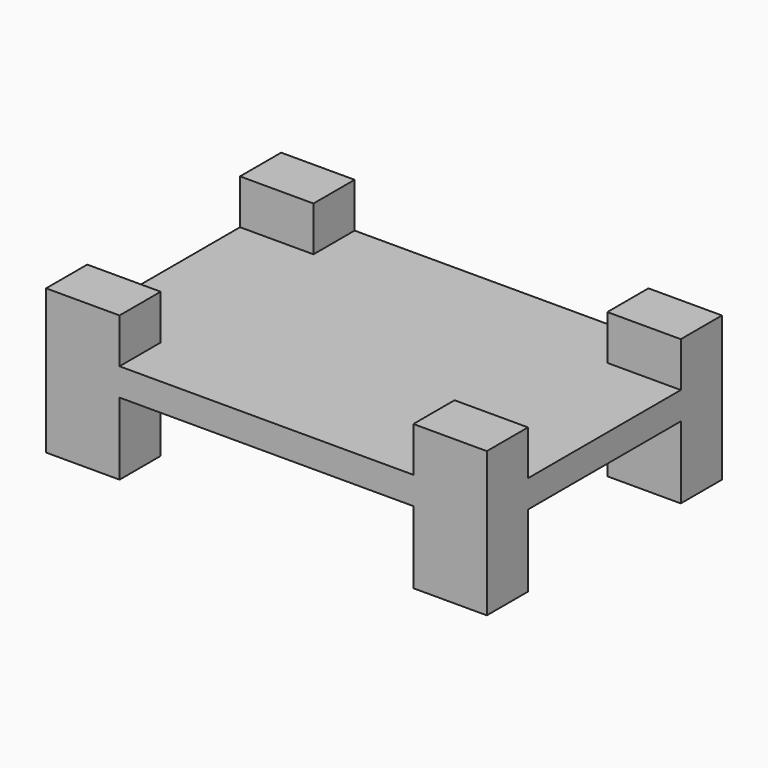
from build123d import *

# Parameters (mm, degrees)
F0_W      = 304.8
F0_H      = 20.32
F1_DEPTH  = 19.05
F2_DEPTH  = 50
F10_DEPTH = 79.4


# Not quite as in the source:
# - a feature names something its author has since deleted; it is built from what else it names


with BuildPart() as f1:
    # F0 (on Top) → F1 (new body)
    with BuildSketch(Plane.XY):
        Rectangle(F0_W, F0_H)
        Polygon((-152.4, 10.16), (152.4, 10.16), (152.4, 66.04), (101.6, 66.04), (101.6, 83.82), (-101.6, 85.344), (-101.6, 66.04), (-152.4, 66.04), align=None)
        Polygon((-101.6, -101.6), (101.6, -101.6), (101.6, -83.82), (-101.6, -85.344), align=None)
        Polygon((101.6, 83.82), (101.6, 101.6), (-101.6, 101.6), (-101.6, 85.344), align=None)
        Polygon((101.6, -66.04), (152.4, -66.04), (152.4, -10.16), (-152.4, -10.16), (-152.4, -66.04), (-101.6, -66.04), (-101.6, -85.344), (101.6, -83.82), align=None)
        Polygon((-152.4, 101.6), (-152.4, 66.04), (-101.6, 66.04), (-101.6, 85.344), (-101.6, 101.6), align=None)
        Polygon((-152.4, -101.6), (-101.6, -101.6), (-101.6, -85.344), (-101.6, -66.04), (-152.4, -66.04), align=None)
        Polygon((101.6, -101.6), (152.4, -101.6), (152.4, -66.04), (101.6, -66.04), (101.6, -83.82), align=None)
        Polygon((101.6, 66.04), (152.4, 66.04), (152.4, 101.6), (101.6, 101.6), (101.6, 83.82), align=None)
    extrude(amount=F1_DEPTH)

    # F0 (on Top) → F2 (join, symmetric)
    with BuildSketch(Plane.XY):
        Polygon((-152.4, -101.6), (-101.6, -101.6), (-101.6, -85.344), (-101.6, -66.04), (-152.4, -66.04), align=None)
        Polygon((-152.4, 101.6), (-152.4, 66.04), (-101.6, 66.04), (-101.6, 85.344), (-101.6, 101.6), align=None)
        Polygon((101.6, 66.04), (152.4, 66.04), (152.4, 101.6), (101.6, 101.6), (101.6, 83.82), align=None)
        Polygon((101.6, -101.6), (152.4, -101.6), (152.4, -66.04), (101.6, -66.04), (101.6, -83.82), align=None)
    extrude(amount=F2_DEPTH, both=True)


with BuildPart() as f7_1:
    # F7: instance of F1
    add(f1.part.mirror(Plane.XZ))


with BuildPart() as f8_1:
    # F8: instance of F7_1
    add(f7_1.part.mirror(Plane.YZ))


with BuildPart() as f8_2:
    # F8: instance of F1
    add(f1.part.mirror(Plane.YZ))


with BuildPart() as f1_1:
    add(f1.part)

    # F9 (on face) → F10 (cut)
    with BuildSketch(Plane.XZ.offset(101.6)):
        with BuildLine():
            ThreePointArc((-28.6936778575, 19.2373767495), (-46.8099126592, 32.3162109562), (-64.9261474609, 19.2373767495))
            Line((-64.9261474609, 19.2373767495), (-28.6936778575, 19.2373767495))
        make_face()
        with BuildLine():
            ThreePointArc((71.8333274126, 19.2373767495), (61.1908975989, 30.3037829778), (50.5484677851, 19.2373767495))
            Line((50.5484677851, 19.2373767495), (71.8333274126, 19.2373767495))
        make_face()
        with BuildLine():
            ThreePointArc((48.6789308488, 19.2373767495), (31.709279865, 31.1125167708), (14.7396288812, 19.2373767495))
            Line((14.7396288812, 19.2373767495), (48.6789308488, 19.2373767495))
        make_face()
        with BuildLine():
            ThreePointArc((11.0462261364, 19.2373767495), (-7.4003641494, 32.1407625343), (-25.8469544351, 19.2373767495))
            Line((-25.8469544351, 19.2373767495), (11.0462261364, 19.2373767495))
        make_face()
    extrude(amount=-F10_DEPTH, mode=Mode.SUBTRACT)


solid = Compound([f7_1.part, f8_1.part, f8_2.part, f1_1.part])
